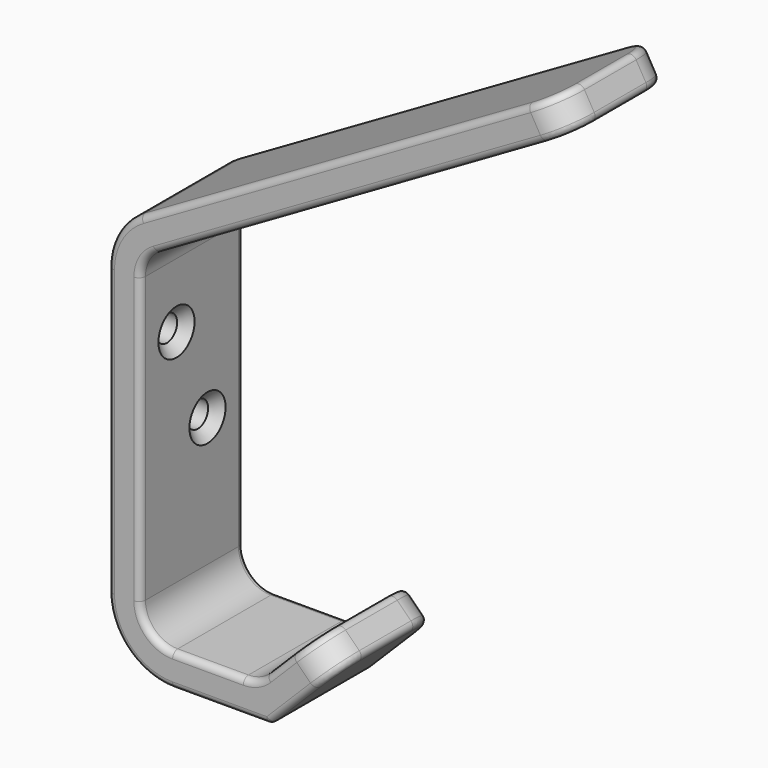
from build123d import *

# Parameters (mm, degrees)
F1_DEPTH        = 20
F2_R            = 5
F3_R            = 5
F4_R            = 10
F5_R            = 5
F6_R            = 5
F7_R            = 5
F8_R            = 5
F9_R            = 5
F10_R           = 1
F11_R           = 1
F12_T1_DEPTH    = 14.5857864376
F12_T3_DEPTH    = 44.2264973081
F12_T5_DEPTH    = 69.2264973081
F12_T7_DEPTH    = 18
F12_T9_DEPTH    = 10
F12_T14_DEPTH   = 1
F12_T20_DEPTH   = 1
F12_T24_ANGLE   = 90
F12_T26_ANGLE   = 90
F12_T28_ANGLE   = 60
F12_T30_ANGLE   = 60
F12_T32_ANGLE   = 90
F12_T34_ANGLE   = 90
F14_D           = 4
F14_CSINK_D     = 7
F14_CSINK_ANGLE = 90
F15_D           = 4
F15_CSINK_D     = 7
F15_CSINK_ANGLE = 90


# Not quite as in the source:
# - a fillet or chamfer that OpenCascade refuses, or shapes differently, is made with other operations: its cross-section is extruded or revolved along the edge and cut away or added


with BuildPart() as f1:
    # F0 (on Front) → F1 (new body)
    with BuildSketch(Plane.XZ):
        Polygon((42.1268583603, 53.609912917), (-27.1551739424, 13.609912917), (-27.1551739424, -46.390087083), (-2.1551739424, -46.390087083), (8.4514277754, -35.7834853652), (4.9158938694, -32.2479514593), (-4.1318040205, -41.2956493492), (-22.1551739424, -41.2956493492), (-22.1551739424, 10.7231615711), (44.6268583603, 49.2797858981), align=None)
    extrude(amount=F1_DEPTH)

    # F2
    f2_edges = [f1.edges().sort_by_distance(p)[0] for p in [
        (-22.155174, -10, -41.295649),
    ]]
    fillet(f2_edges, radius=F2_R)

    # F3
    f3_edges = [f1.edges().sort_by_distance(p)[0] for p in [
        (-4.131804, -10, -41.295649),
    ]]
    fillet(f3_edges, radius=F3_R)

    # F4
    f4_edges = [f1.edges().sort_by_distance(p)[0] for p in [
        (-27.155174, -10, -46.390087),
        (-27.155174, -10, 13.609913),
    ]]
    fillet(f4_edges, radius=F4_R)

    # F5
    f5_edges = [f1.edges().sort_by_distance(p)[0] for p in [
        (-22.155174, -10, 10.723162),
    ]]
    fillet(f5_edges, radius=F5_R)

    # F6
    f6_edges = [f1.edges().sort_by_distance(p)[0] for p in [
        (6.683661, 0, -34.015718),
    ]]
    fillet(f6_edges, radius=F6_R)

    # F7
    f7_edges = [f1.edges().sort_by_distance(p)[0] for p in [
        (6.683661, -20, -34.015718),
    ]]
    fillet(f7_edges, radius=F7_R)

    # F8
    f8_edges = [f1.edges().sort_by_distance(p)[0] for p in [
        (43.376858, -20, 51.444849),
    ]]
    fillet(f8_edges, radius=F8_R)

    # F9
    f9_edges = [f1.edges().sort_by_distance(p)[0] for p in [
        (43.376858, 0, 51.444849),
    ]]
    fillet(f9_edges, radius=F9_R)

    # F10
    f10_edges = [f1.edges().sort_by_distance(p)[0] for p in [
        (43.358594, -18.535534, 48.547553),
    ]]
    fillet(f10_edges, radius=F10_R)

    # F11
    f11_edges = [f1.edges().sort_by_distance(p)[0] for p in [
        (7.415894, -18.535534, -36.819019),
    ]]
    fillet(f11_edges, radius=F11_R)

    # F12: fillet of radius 1 on 14 edges, made by hand

    # F12_s2 → F12_t1 (cut)
    with BuildSketch(Plane.YZ.offset(-17.1551739424)):
        with BuildLine():
            ThreePointArc((0, -45.390087083), (-0.2928932188, -46.0971938642), (-1, -46.390087083))
            Line((-1, -46.390087083), (0, -46.390087083))
            Line((0, -46.390087083), (0, -45.390087083))
        make_face()
        with BuildLine():
            ThreePointArc((-19, -46.390087083), (-19.7071067812, -46.0971938642), (-20, -45.390087083))
            Line((-20, -45.390087083), (-20, -46.390087083))
            Line((-20, -46.390087083), (-19, -46.390087083))
        make_face()
    extrude(amount=F12_T1_DEPTH, mode=Mode.SUBTRACT)

    # F12_s4 → F12_t3 (cut)
    with BuildSketch(Plane.XY.offset(-36.390087083)):
        with BuildLine():
            ThreePointArc((-26.1551739424, 0), (-26.8622807236, -0.2928932188), (-27.1551739424, -1))
            Line((-27.1551739424, -1), (-27.1551739424, 0))
            Line((-27.1551739424, 0), (-26.1551739424, 0))
        make_face()
        with BuildLine():
            ThreePointArc((-27.1551739424, -19), (-26.8622807236, -19.7071067812), (-26.1551739424, -20))
            Line((-26.1551739424, -20), (-27.1551739424, -20))
            Line((-27.1551739424, -20), (-27.1551739424, -19))
        make_face()
    extrude(amount=F12_T3_DEPTH, mode=Mode.SUBTRACT)

    # F12_s6 → F12_t5 (cut)
    with BuildSketch(Plane(origin=(50.4787899917, 0, 29.1439429901), x_dir=(0, 1, 0), z_dir=(-0.8660254038, 0, -0.5))):
        with BuildLine():
            ThreePointArc((0, -24.3641173007), (-0.2928932188, -25.0712240818), (-1, -25.3641173007))
            Line((-1, -25.3641173007), (0, -25.3641173007))
            Line((0, -25.3641173007), (0, -24.3641173007))
        make_face()
        with BuildLine():
            ThreePointArc((-19, -25.3641173007), (-19.7071067812, -25.0712240818), (-20, -24.3641173007))
            Line((-20, -24.3641173007), (-20, -25.3641173007))
            Line((-20, -25.3641173007), (-19, -25.3641173007))
        make_face()
    extrude(amount=F12_T5_DEPTH, mode=Mode.SUBTRACT)

    # F12_s8 → F12_t7 (cut)
    with BuildSketch(Plane.XZ.offset(1)):
        with BuildLine():
            ThreePointArc((-2.5693875048, -46.390087083), (-2.1867040725, -46.3139666155), (-1.8622807236, -46.0971938642))
            Line((-1.8622807236, -46.0971938642), (-2.1551739424, -46.390087083))
            Line((-2.1551739424, -46.390087083), (-2.5693875048, -46.390087083))
        make_face()
    extrude(amount=F12_T7_DEPTH, mode=Mode.SUBTRACT)

    # F12_s10 → F12_t9 (cut)
    with BuildSketch(Plane.XZ.offset(5)):
        with BuildLine():
            ThreePointArc((41.2608329565, 53.109912917), (42.0196520016, 53.2098133395), (42.6268583603, 52.7438875132))
            Line((42.6268583603, 52.7438875132), (42.1268583603, 53.609912917))
            Line((42.1268583603, 53.609912917), (41.2608329565, 53.109912917))
        make_face()
    extrude(amount=F12_T9_DEPTH, mode=Mode.SUBTRACT)


with BuildPart() as f12_tool12:
    # F12_s13 → F12_t14 (new body)
    with BuildSketch(Plane.XZ.offset(19)):
        Polygon((-2.5693875048, -45.390087083), (-1.8622807236, -46.0971938642), (-2.1551739424, -46.390087083), (-2.5693875048, -46.390087083), align=None)
    extrude(amount=F12_T14_DEPTH)

    # F12_s15 → F12_t16 (revolve, cut)
    with BuildSketch(Plane(origin=(-2.5693875048, -19, -45.390087083), x_dir=(-0.3826834324, 0, 0.9238795325), z_dir=(0.9238795325, 0, 0.3826834324))):
        with BuildLine():
            ThreePointArc((0, -1), (1, 0), (0, 1))
            Line((0, 1), (0, -1))
        make_face()
    revolve(axis=Axis((-2.5693875048, -19, -45.390087083), (0, -1, 0)), mode=Mode.SUBTRACT)


with BuildPart() as f1_1:
    add(f1.part)

    # F12_t11: cut F12_tool12
    add(f12_tool12.part, mode=Mode.SUBTRACT)


with BuildPart() as f12_tool18:
    # F12_s19 → F12_t20 (new body)
    with BuildSketch(Plane.XZ.offset(1)):
        Polygon((-2.5693875048, -45.390087083), (-1.8622807236, -46.0971938642), (-2.1551739424, -46.390087083), (-2.5693875048, -46.390087083), align=None)
    extrude(amount=-F12_T20_DEPTH)

    # F12_s21 → F12_t22 (revolve, cut)
    with BuildSketch(Plane(origin=(-2.5693875048, -1, -45.390087083), x_dir=(-0.3826834324, 0, 0.9238795325), z_dir=(-0.9238795325, 0, -0.3826834324))):
        with BuildLine():
            ThreePointArc((0, -1), (1, 0), (0, 1))
            Line((0, 1), (0, -1))
        make_face()
    revolve(axis=Axis((-2.5693875048, -1, -45.390087083), (0, 1, 0)), mode=Mode.SUBTRACT)


with BuildPart() as f1_2:
    add(f1_1.part)

    # F12_t17: cut F12_tool18
    add(f12_tool18.part, mode=Mode.SUBTRACT)

    # F12_s23 → F12_t24 (revolve, cut)
    with BuildSketch(Plane.YZ.offset(-17.1551739424)):
        with BuildLine():
            ThreePointArc((-19, -46.390087083), (-19.7071067812, -46.0971938642), (-20, -45.390087083))
            Line((-20, -45.390087083), (-20, -46.390087083))
            Line((-20, -46.390087083), (-19, -46.390087083))
        make_face()
    revolve(axis=Axis((-17.1551739424, -20, -36.390087083), (0, 1, 0)), revolution_arc=F12_T24_ANGLE, mode=Mode.SUBTRACT)

    # F12_s25 → F12_t26 (revolve, cut)
    with BuildSketch(Plane.YZ.offset(-17.1551739424)):
        with BuildLine():
            ThreePointArc((0, -45.390087083), (-0.2928932188, -46.0971938642), (-1, -46.390087083))
            Line((-1, -46.390087083), (0, -46.390087083))
            Line((0, -46.390087083), (0, -45.390087083))
        make_face()
    revolve(axis=Axis((-17.1551739424, 0, -36.390087083), (0, 1, 0)), revolution_arc=F12_T26_ANGLE, mode=Mode.SUBTRACT)

    # F12_s27 → F12_t28 (revolve, cut)
    with BuildSketch(Plane(origin=(-9.4731152921, 0, -5.469305664), x_dir=(0, 1, 0), z_dir=(0.8660254038, 0, 0.5))):
        with BuildLine():
            ThreePointArc((0, 24.3641173007), (-0.2928932188, 25.0712240818), (-1, 25.3641173007))
            Line((-1, 25.3641173007), (0, 25.3641173007))
            Line((0, 25.3641173007), (0, 24.3641173007))
        make_face()
    revolve(axis=Axis((-17.1551739424, 0, 7.8364102251), (0, -1, 0)), revolution_arc=F12_T28_ANGLE, mode=Mode.SUBTRACT)

    # F12_s29 → F12_t30 (revolve, cut)
    with BuildSketch(Plane(origin=(-9.4731152921, 0, -5.469305664), x_dir=(0, 1, 0), z_dir=(0.8660254038, 0, 0.5))):
        with BuildLine():
            ThreePointArc((-19, 25.3641173007), (-19.7071067812, 25.0712240818), (-20, 24.3641173007))
            Line((-20, 24.3641173007), (-20, 25.3641173007))
            Line((-20, 25.3641173007), (-19, 25.3641173007))
        make_face()
    revolve(axis=Axis((-17.1551739424, -20, 7.8364102251), (0, -1, 0)), revolution_arc=F12_T30_ANGLE, mode=Mode.SUBTRACT)

    # F12_s31 → F12_t32 (revolve, cut)
    with BuildSketch(Plane.XZ.offset(5)):
        with BuildLine():
            ThreePointArc((41.2608329565, 53.109912917), (42.0196520016, 53.2098133395), (42.6268583603, 52.7438875132))
            Line((42.6268583603, 52.7438875132), (42.1268583603, 53.609912917))
            Line((42.1268583603, 53.609912917), (41.2608329565, 53.109912917))
        make_face()
    revolve(axis=Axis((37.7967313414, -5, 51.109912917), (-0.5, 0, 0.8660254038)), revolution_arc=F12_T32_ANGLE, mode=Mode.SUBTRACT)

    # F12_s33 → F12_t34 (revolve, cut)
    with BuildSketch(Plane(origin=(50.4787899917, 0, 29.1439429901), x_dir=(0, 1, 0), z_dir=(-0.8660254038, 0, -0.5))):
        with BuildLine():
            ThreePointArc((-19, -25.3641173007), (-19.7071067812, -25.0712240818), (-20, -24.3641173007))
            Line((-20, -24.3641173007), (-20, -25.3641173007))
            Line((-20, -25.3641173007), (-19, -25.3641173007))
        make_face()
    revolve(axis=Axis((37.7967313414, -15, 51.109912917), (-0.5, 0, 0.8660254038)), revolution_arc=F12_T34_ANGLE, mode=Mode.SUBTRACT)

    # F14 (through all)
    with Locations(Plane.YZ.offset(-22.1551739424)):
        with Locations((-13, -2.1635897749)):
            CounterSinkHole(F14_D / 2, F14_CSINK_D / 2, counter_sink_angle=F14_CSINK_ANGLE)

    # F15 (through all)
    with Locations(Plane.YZ.offset(-22.1551739424)):
        with Locations((-7, -16.2956493492)):
            CounterSinkHole(F15_D / 2, F15_CSINK_D / 2, counter_sink_angle=F15_CSINK_ANGLE)


solid = f1_2.part
